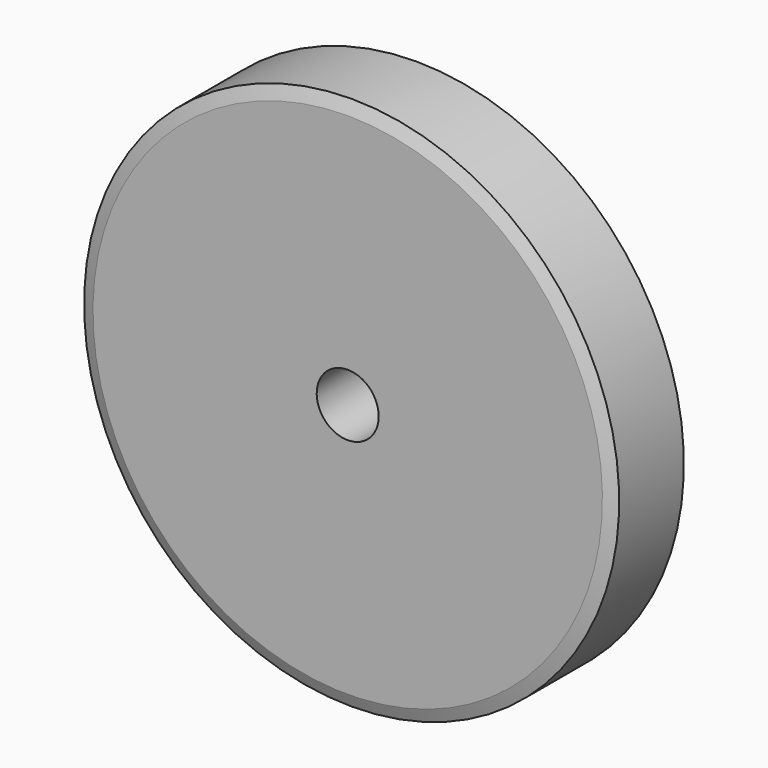
from build123d import *

# Parameters (mm, degrees)
F0_W        = 117
F0_H        = 154.5
F0_H_2      = 150.5
F0_W_2      = 67.4791876724
F2_R        = 1.5875
F3_SIZE     = 0.7696969697
F4_C1_SIZE2 = 6.35
F4_C1_SIZE  = 16.51
F4_C2_SIZE2 = 16.51
F4_C2_SIZE  = 6.35


with BuildPart() as f1:
    # F0 (on Right) → F1 (revolve)
    with BuildSketch(Plane.YZ):
        with Locations((58.5, 267.75)):
            Rectangle(F0_W, F0_H)
        with Locations((58.5, 115.25)):
            Rectangle(F0_W, F0_H_2)
        with Locations((150.7395938362, 115.25)):
            Rectangle(F0_W_2, F0_H_2)
    revolve(axis=Axis((0, 115.410885826, 0), (0, 1, 0)))

    # F2
    f2_edges = [f1.edges().sort_by_distance(p)[0] for p in [
        (0, 117, -190.5),
    ]]
    fillet(f2_edges, radius=F2_R)

    # F3
    f3_edges = [f1.edges().sort_by_distance(p)[0] for p in [
        (0, 184.479188, -190.5),
    ]]
    chamfer(f3_edges, length=F3_SIZE)

    # F4: chamfer of 6.35 x 16.51 on 4 edges, made by hand

    # F4_c1
    f4_c1_edges = [f1.edges().sort_by_distance(p)[0] for p in [
        (0, 117, -345),
    ]]
    f4_c1_side = f1.faces().sort_by_distance((0, 117, -344.873))[0]
    chamfer(f4_c1_edges, length=F4_C1_SIZE, length2=F4_C1_SIZE2, reference=f4_c1_side)

    # F4_c2
    f4_c2_edges = [f1.edges().sort_by_distance(p)[0] for p in [
        (0, 0, -345),
    ]]
    f4_c2_side = f1.faces().sort_by_distance((0, 0.127, -345))[0]
    chamfer(f4_c2_edges, length=F4_C2_SIZE, length2=F4_C2_SIZE2, reference=f4_c2_side)


solid = f1.part
